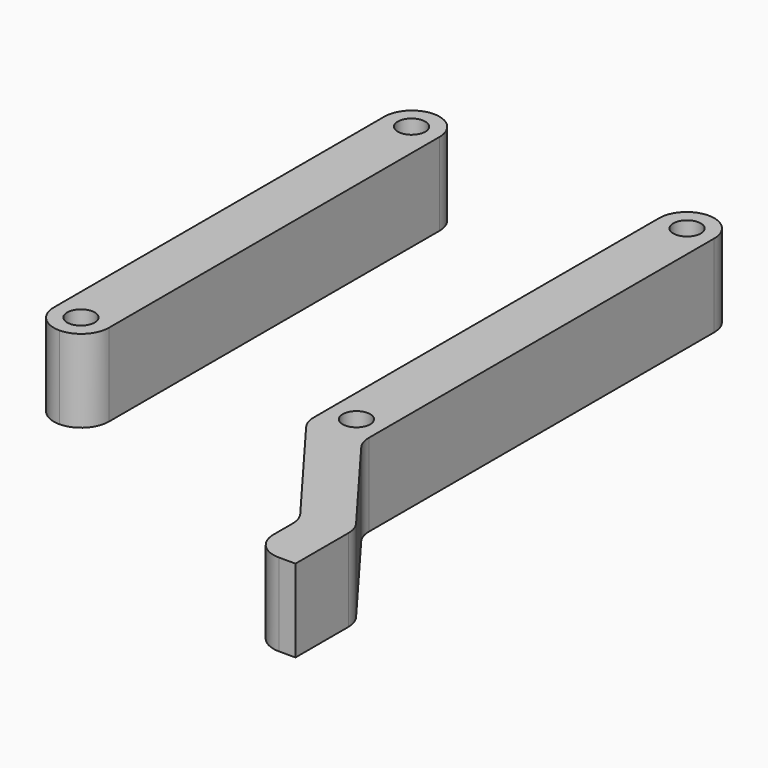
from build123d import *

# Parameters (mm, degrees)
F0_W     = 10
F0_H     = 85
F0_R     = 2.5
F1_DEPTH = 15
F5_DEPTH = 15
F6_R     = 4.99999
F6_2_R   = 4.99999


# Not quite as in the source:
# - a fillet or chamfer is up to 0.001 mm smaller than in the source, because OpenCascade refuses the exact size


with BuildPart() as f1:
    # F0 (on Top) → F1 (new body)
    with BuildSketch(Plane.XY):
        with Locations((0.0677526742, 37.5)):
            Rectangle(F0_W, F0_H)
        Circle(F0_R, mode=Mode.SUBTRACT)
        with Locations((0, 75)):
            Circle(F0_R, mode=Mode.SUBTRACT)
    extrude(amount=F1_DEPTH)


with BuildPart() as f3_1:
    # F3: instance of F1
    add(f1.part.mirror(Plane.YZ.offset(25)))

    # F4 (on Top) → F5 (join)
    with BuildSketch(Plane.XY):
        Polygon((54.9322473258, -5), (44.9322473258, -5), (62.9322473258, -29), (62.9322473258, -40), (70.9322473258, -40), (70.9322473258, -26.3333333333), align=None)
    extrude(amount=F5_DEPTH)

    # F6#2 (radius 5 in the source; OpenCascade refuses exactly that, so slightly less here)
    f6_2_edges = [f3_1.edges().sort_by_distance(p)[0] for p in [
        (44.932247, -5, 7.5),
        (70.932247, -26.333333, 7.5),
        (62.932247, -29, 7.5),
        (54.932247, -5, 7.5),
        (54.932247, 80, 7.5),
        (44.932247, 80, 7.5),
        (62.932247, -40, 7.5),
    ]]
    fillet(f6_2_edges, radius=F6_2_R)


with BuildPart() as f1_1:
    add(f1.part)

    # F6 (radius 5 in the source; OpenCascade refuses exactly that, so slightly less here)
    f6_edges = [f1_1.edges().sort_by_distance(p)[0] for p in [
        (5.067753, -5, 7.5),
        (-4.932247, -5, 7.5),
        (5.067753, 80, 7.5),
        (-4.932247, 80, 7.5),
    ]]
    fillet(f6_edges, radius=F6_R)


solid = Compound([f3_1.part, f1_1.part])
